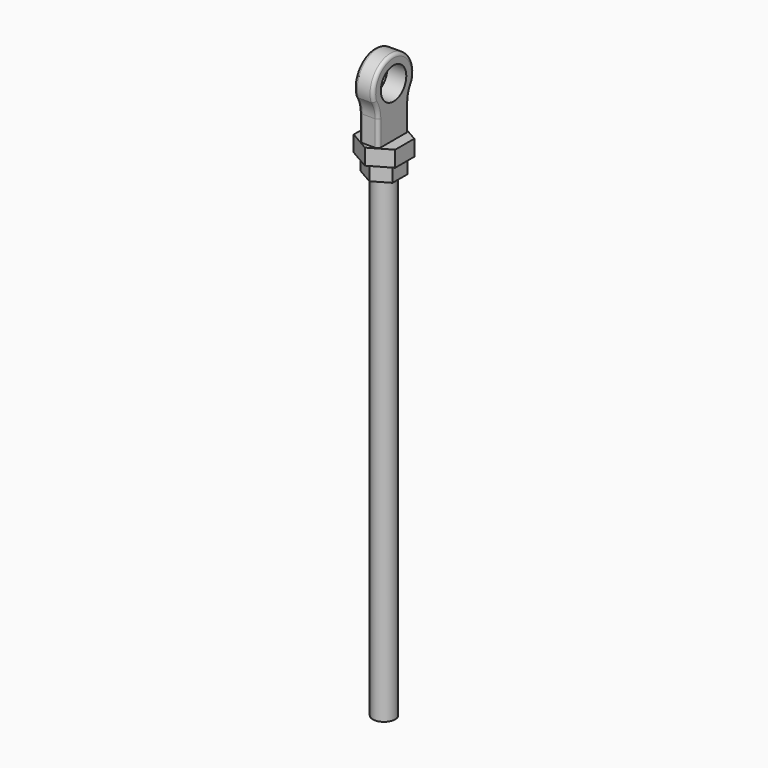
from build123d import *

# Parameters (mm, degrees)
F0_R         = 3.5
F1_DEPTH     = 150
F3_DEPTH     = 5
F5_DEPTH     = 5
F6_R         = 5
F7_DEPTH     = 3
F8_F1_R      = 1
F8_F2_R      = 1
F8_T3_DEPTH  = 8
F8_T6_ANGLE  = 74.8218835265
F8_T7_DEPTH  = 8
F8_T10_ANGLE = 74.8218835265
F8_T11_DEPTH = 8
F8_T14_ANGLE = 74.8218835265
F8_T15_DEPTH = 8
F8_T18_ANGLE = 74.8218835265


# Not quite as in the source:
# - a fillet or chamfer that OpenCascade refuses, or shapes differently, is made with other operations: its cross-section is extruded or revolved along the edge and cut away or added


with BuildPart() as f1:
    # F0 (on Top) → F1 (new body)
    with BuildSketch(Plane.XY):
        Circle(F0_R)
    extrude(amount=F1_DEPTH)

    # F2 (on face) → F3 (join)
    with BuildSketch(Plane.XY.offset(150)):
        Polygon((5, -2.8867513459), (5, 2.8867513459), (0, 5.7735026919), (-5, 2.8867513459), (-5, -2.8867513459), (0, -5.7735026919), align=None)
    extrude(amount=F3_DEPTH)

    # F4 (on face) → F5 (join)
    with BuildSketch(Plane.XY.offset(155)):
        Polygon((6.5, -3.7527767497), (6.5, 3.7527767497), (0, 7.5055534995), (-6.5, 3.7527767497), (-6.5, -3.7527767497), (0, -7.5055534995), align=None)
    extrude(amount=F5_DEPTH)

    # F6 (on Right) → F7 (join, symmetric)
    with BuildSketch(Plane.YZ):
        with BuildLine():
            ThreePointArc((6, 168), (6.4085678246, 170.709769965), (7.5979446603, 173.1786084922))
            ThreePointArc((7.5979446603, 173.1786084922), (0, 183.6828522781), (-7.5979446603, 173.1786084922))
            ThreePointArc((-7.5979446603, 173.1786084922), (-6.4085678246, 170.709769965), (-6, 168))
            Line((-6, 168), (-6, 160))
            Line((-6, 160), (0, 160))
            Line((0, 160), (6, 160))
            Line((6, 160), (6, 168))
        make_face()
        with Locations((0, 175.6828522781)):
            Circle(F6_R, mode=Mode.SUBTRACT)
    extrude(amount=F7_DEPTH, both=True)

    # F8: fillet of radius 1 on 10 edges, made by hand

    # F8_f1
    f8_f1_edges = [f1.edges().sort_by_distance(p)[0] for p in [
        (3, 0, 183.6828522781),
    ]]
    fillet(f8_f1_edges, radius=F8_F1_R)

    # F8_f2
    f8_f2_edges = [f1.edges().sort_by_distance(p)[0] for p in [
        (-3, 0, 183.6828522781),
    ]]
    fillet(f8_f2_edges, radius=F8_F2_R)

    # F8_s4 → F8_t3 (cut)
    with BuildSketch(Plane.XY.offset(160)):
        with BuildLine():
            ThreePointArc((3, 5), (2.7071067812, 5.7071067812), (2, 6))
            Line((2, 6), (2, 6.02))
            Line((2, 6.02), (3.02, 6.02))
            Line((3.02, 6.02), (3.02, 5))
            Line((3.02, 5), (3, 5))
        make_face()
    extrude(amount=F8_T3_DEPTH, mode=Mode.SUBTRACT)

    # F8_s5 → F8_t6 (revolve, cut)
    with BuildSketch(Plane.XY.offset(168)):
        with BuildLine():
            ThreePointArc((2, 6), (2.7071067812, 5.7071067812), (3, 5))
            Line((3, 5), (3.02, 5))
            Line((3.02, 5), (3.02, 6.02))
            Line((3.02, 6.02), (2, 6.02))
            Line((2, 6.02), (2, 6))
        make_face()
    revolve(axis=Axis((3, 15.190372415, 168), (-1, 0, 0)), revolution_arc=F8_T6_ANGLE, mode=Mode.SUBTRACT)

    # F8_s8 → F8_t7 (cut)
    with BuildSketch(Plane.XY.offset(160)):
        with BuildLine():
            ThreePointArc((-2, 6), (-2.7071067812, 5.7071067812), (-3, 5))
            Line((-3, 5), (-3.02, 5))
            Line((-3.02, 5), (-3.02, 6.02))
            Line((-3.02, 6.02), (-2, 6.02))
            Line((-2, 6.02), (-2, 6))
        make_face()
    extrude(amount=F8_T7_DEPTH, mode=Mode.SUBTRACT)

    # F8_s9 → F8_t10 (revolve, cut)
    with BuildSketch(Plane.XY.offset(168)):
        with BuildLine():
            ThreePointArc((-2, 6), (-2.7071067812, 5.7071067812), (-3, 5))
            Line((-3, 5), (-3.02, 5))
            Line((-3.02, 5), (-3.02, 6.02))
            Line((-3.02, 6.02), (-2, 6.02))
            Line((-2, 6.02), (-2, 6))
        make_face()
    revolve(axis=Axis((-3, 15.190372415, 168), (-1, 0, 0)), revolution_arc=F8_T10_ANGLE, mode=Mode.SUBTRACT)

    # F8_s12 → F8_t11 (cut)
    with BuildSketch(Plane.XY.offset(160)):
        with BuildLine():
            ThreePointArc((-2, -6), (-2.7071067812, -5.7071067812), (-3, -5))
            Line((-3, -5), (-3.02, -5))
            Line((-3.02, -5), (-3.02, -6.02))
            Line((-3.02, -6.02), (-2, -6.02))
            Line((-2, -6.02), (-2, -6))
        make_face()
    extrude(amount=F8_T11_DEPTH, mode=Mode.SUBTRACT)

    # F8_s13 → F8_t14 (revolve, cut)
    with BuildSketch(Plane(origin=(0, -56.6005519955, 15.3548182499), x_dir=(1, 0, 0), z_dir=(0, -0.9651165645, 0.2618205815))):
        with BuildLine():
            ThreePointArc((-2, 167.3528031133), (-2.7071067812, 167.6456963322), (-3, 168.3528031133))
            Line((-3, 168.3528031133), (-3.02, 168.3528031133))
            Line((-3.02, 168.3528031133), (-3.02, 167.3328031133))
            Line((-3.02, 167.3328031133), (-2, 167.3328031133))
            Line((-2, 167.3328031133), (-2, 167.3528031133))
        make_face()
    revolve(axis=Axis((-3, -15.190372415, 168), (-1, 0, 0)), revolution_arc=F8_T14_ANGLE, mode=Mode.SUBTRACT)

    # F8_s16 → F8_t15 (cut)
    with BuildSketch(Plane.XY.offset(160)):
        with BuildLine():
            ThreePointArc((2, -6), (2.7071067812, -5.7071067812), (3, -5))
            Line((3, -5), (3.02, -5))
            Line((3.02, -5), (3.02, -6.02))
            Line((3.02, -6.02), (2, -6.02))
            Line((2, -6.02), (2, -6))
        make_face()
    extrude(amount=F8_T15_DEPTH, mode=Mode.SUBTRACT)

    # F8_s17 → F8_t18 (revolve, cut)
    with BuildSketch(Plane(origin=(0, -56.6005519955, 15.3548182499), x_dir=(1, 0, 0), z_dir=(0, -0.9651165645, 0.2618205815))):
        with BuildLine():
            ThreePointArc((2, 167.3528031133), (2.7071067812, 167.6456963322), (3, 168.3528031133))
            Line((3, 168.3528031133), (3.02, 168.3528031133))
            Line((3.02, 168.3528031133), (3.02, 167.3328031133))
            Line((3.02, 167.3328031133), (2, 167.3328031133))
            Line((2, 167.3328031133), (2, 167.3528031133))
        make_face()
    revolve(axis=Axis((3, -15.190372415, 168), (-1, 0, 0)), revolution_arc=F8_T18_ANGLE, mode=Mode.SUBTRACT)


solid = f1.part
